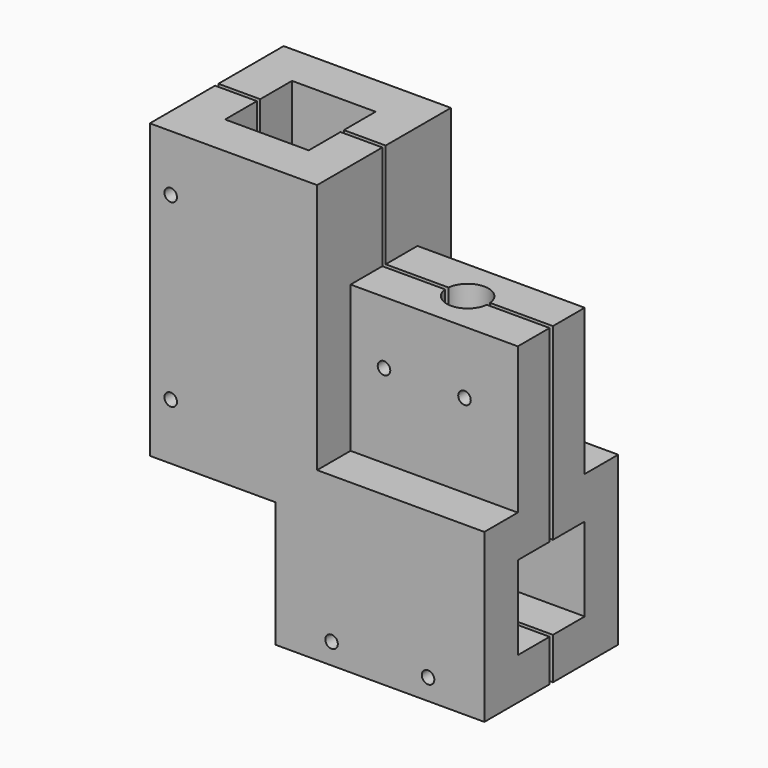
from build123d import *

# Parameters (mm, degrees)
F1_DEPTH        = 20
F2_W            = 50
F2_H            = 10
F3_DEPTH        = 10
F4_W            = 50
F4_H            = 10
F5_DEPTH        = 10
F6_W            = 50
F6_H            = 10
F7_DEPTH        = 30
F8_W            = 10
F8_H            = 10
F9_DEPTH        = 60
F10_W           = 10
F10_H           = 70
F11_DEPTH       = 30
F12_R           = 5
F13_DEPTH       = 15
F16_DEPTH       = 70
F17_T1_DEPTH    = 17.2150489639
F17_S1_T1_DEPTH = 10.5
F18_W           = 10
F18_H           = 70
F18_W_2         = 50
F18_H_2         = 10
F20_DEPTH       = 9.5
F19_W           = 10
F19_H           = 70
F19_W_2         = 50
F19_H_2         = 10
F21_DEPTH       = 9.5
F22_R           = 1.5
F23_DEPTH       = 20
F24_R           = 1.5
F25_DEPTH       = 20
F26_DEPTH       = 3
F28_R           = 1.5
F29_DEPTH       = 10
F27_R           = 1.5
F30_DEPTH       = 10
F31_DEPTH       = 3


# Not quite as in the source:
# - a fillet or chamfer that OpenCascade refuses, or shapes differently, is made with other operations: its cross-section is extruded or revolved along the edge and cut away or added


with BuildPart() as f1:
    # F0 (on Front) → F1 (new body)
    with BuildSketch(Plane.XZ):
        Polygon((-40, 89.1929870069), (-50, 89.1929870069), (-50, 19.1929870069), (0, 19.1929870069), (0, 64.1929870069), (-40, 64.1929870069), align=None)
    extrude(amount=F1_DEPTH)

    # F2 (on face) → F3 (join)
    with BuildSketch(Plane.XZ.offset(20)):
        with Locations((-25, 24.1929870069)):
            Rectangle(F2_W, F2_H)
    extrude(amount=F3_DEPTH)

    # F4 (on face) → F5 (join)
    with BuildSketch(Plane(origin=(0, 0, 0), x_dir=(-1, 0, 0), z_dir=(0, 1, 0))):
        with Locations((25, 24.1929870069)):
            Rectangle(F4_W, F4_H)
    extrude(amount=F5_DEPTH)

    # F6 (on face) → F7 (join)
    with BuildSketch(Plane(origin=(0, 0, 19.1929870069), x_dir=(1, 0, 0), z_dir=(0, 0, -1))):
        with Locations((-25, 25)):
            Rectangle(F6_W, F6_H)
        with Locations((-25, -5)):
            Rectangle(F6_W, F6_H)
    extrude(amount=F7_DEPTH)

    # F8 (on face) → F9 (join)
    with BuildSketch(Plane.XY.offset(29.1929870069)):
        with Locations((-45, 5)):
            Rectangle(F8_W, F8_H)
        with Locations((-45, -25)):
            Rectangle(F8_W, F8_H)
    extrude(amount=F9_DEPTH)

    # F10 (on face) → F11 (join)
    with BuildSketch(Plane(origin=(-50, 0, 0), x_dir=(0, -1, 0), z_dir=(-1, 0, 0))):
        with Locations((25, 54.1929870069)):
            Rectangle(F10_W, F10_H)
        with Locations((-5, 54.1929870069)):
            Rectangle(F10_W, F10_H)
    extrude(amount=F11_DEPTH)

    # F12 (on face) → F13 (cut)
    with BuildSketch(Plane.XY.offset(64.1929870069)):
        with Locations((-20, -10)):
            Circle(F12_R)
    extrude(amount=-F13_DEPTH, mode=Mode.SUBTRACT)

    # F15 (on face) + F14 (on face) → F16 (cut)
    with BuildSketch(Plane.XY.offset(64.1929870069)):
        with BuildLine():
            Line((0, -10.5), (0, -9.5))
            Line((0, -9.5), (-15.0250628145, -9.5))
            ThreePointArc((-15.0250628145, -9.5), (-15.0062696344, -9.7496861247), (-15, -10))
            ThreePointArc((-15, -10), (-15.0062696344, -10.2503138753), (-15.0250628145, -10.5))
            Line((-15.0250628145, -10.5), (0, -10.5))
        make_face()
        with BuildLine():
            Line((-15.0250628145, -9.5), (-24.9749371855, -9.5))
            ThreePointArc((-24.9749371855, -9.5), (-25, -10), (-24.9749371855, -10.5))
            Line((-24.9749371855, -10.5), (-15.0250628145, -10.5))
            ThreePointArc((-15.0250628145, -10.5), (-15.0062696344, -10.2503138753), (-15, -10))
            ThreePointArc((-15, -10), (-15.0062696344, -9.7496861247), (-15.0250628145, -9.5))
        make_face()
        with BuildLine():
            Line((-24.9749371855, -9.5), (-40, -9.5))
            Line((-40, -9.5), (-40, -10.5))
            Line((-40, -10.5), (-24.9749371855, -10.5))
            ThreePointArc((-24.9749371855, -10.5), (-25, -10), (-24.9749371855, -9.5))
        make_face()
    with BuildSketch(Plane.XY.offset(89.1929870069)):
        Polygon((-40, -10.5), (-40, -10), (-40, -9.5), (-50, -9.5), (-50, -10.5), align=None)
    extrude(amount=-F16_DEPTH, mode=Mode.SUBTRACT)

    # F17: chamfer of 3 on 1 edges, made by hand

    # F17_s2 → F17_t1 (cut)
    with BuildSketch(Plane.XZ.offset(2.7849510361)):
        Polygon((-47, 19.1929870069), (-50, 22.1929870069), (-50, 19.1929870069), align=None)
    extrude(amount=F17_T1_DEPTH, mode=Mode.SUBTRACT)

    # F17#s1: chamfer of 3 on 1 edges, made by hand

    # F17_s1_s2 → F17_s1_t1 (cut)
    with BuildSketch(Plane.XZ):
        Polygon((-50, 22.1929870069), (-47, 19.1929870069), (-50, 19.1929870069), align=None)
    extrude(amount=F17_S1_T1_DEPTH, mode=Mode.SUBTRACT)

    # F18 (on face) → F20 (join)
    with BuildSketch(Plane.XZ):
        with Locations((-75, 54.1929870069)):
            Rectangle(F18_W, F18_H)
        with Locations((-25, -5.8070129931)):
            Rectangle(F18_W_2, F18_H_2)
    extrude(amount=F20_DEPTH)

    # F19 (on face) → F21 (join)
    with BuildSketch(Plane(origin=(0, -20, 0), x_dir=(-1, 0, 0), z_dir=(0, 1, 0))):
        with Locations((75, 54.1929870069)):
            Rectangle(F19_W, F19_H)
        with Locations((25, -5.8070129931)):
            Rectangle(F19_W_2, F19_H_2)
    extrude(amount=F21_DEPTH)

    # F22 (on face) → F23 (cut)
    with BuildSketch(Plane.XZ.offset(30)):
        with Locations((-13.464, -5.8070129931)):
            Circle(F22_R)
        with Locations((-75, 75.7289870069)):
            Circle(F22_R)
        with Locations((-75, 32.6569870069)):
            Circle(F22_R)
        with Locations((-36.536, -5.8070129931)):
            Circle(F22_R)
    extrude(amount=-F23_DEPTH, mode=Mode.SUBTRACT)

    # F24 (on face) → F25 (cut)
    with BuildSketch(Plane(origin=(0, 10, 0), x_dir=(-1, 0, 0), z_dir=(0, 1, 0))):
        with Locations((13.4641016151, -5.8070129931)):
            Circle(F24_R)
        with Locations((36.5358983849, -5.8070129931)):
            Circle(F24_R)
        with Locations((75, 32.657088622)):
            Circle(F24_R)
        with Locations((75, 75.7288853918)):
            Circle(F24_R)
    extrude(amount=-F25_DEPTH, mode=Mode.SUBTRACT)

    # F24 (on face) → F26 (cut)
    with BuildSketch(Plane(origin=(0, 10, 0), x_dir=(-1, 0, 0), z_dir=(0, 1, 0))):
        Polygon((34.8038475773, -2.8070129931), (33.0717967697, -5.8070129931), (34.8038475773, -8.8070129931), (38.2679491924, -8.8070129931), (40, -5.8070129931), (38.2679491924, -2.8070129931), align=None)
        with Locations((36.5358983849, -5.8070129931)):
            Circle(F24_R, mode=Mode.SUBTRACT)
        Polygon((11.7320508076, -2.8070129931), (10, -5.8070129931), (11.7320508076, -8.8070129931), (15.1961524227, -8.8070129931), (16.9282032303, -5.8070129931), (15.1961524227, -2.8070129931), align=None)
        with Locations((13.4641016151, -5.8070129931)):
            Circle(F24_R, mode=Mode.SUBTRACT)
        Polygon((72, 30.9250378145), (75, 29.1929870069), (78, 30.9250378145), (78, 34.3891394296), (75, 36.1211902372), (72, 34.3891394296), align=None)
        with Locations((75, 32.657088622)):
            Circle(F24_R, mode=Mode.SUBTRACT)
        Polygon((72, 73.9968345842), (75, 72.2647837766), (78, 73.9968345842), (78, 77.4609361993), (75, 79.1929870069), (72, 77.4609361993), align=None)
        with Locations((75, 75.7288853918)):
            Circle(F24_R, mode=Mode.SUBTRACT)
    extrude(amount=-F26_DEPTH, mode=Mode.SUBTRACT)

    # F28 (on face) → F29 (cut)
    with BuildSketch(Plane(origin=(0, 0, 0), x_dir=(-1, 0, 0), z_dir=(0, 1, 0))):
        with Locations((32, 49.1929870069)):
            Circle(F28_R)
        with Locations((12.75, 49.1929870069)):
            Circle(F28_R)
    extrude(amount=-F29_DEPTH, mode=Mode.SUBTRACT)

    # F27 (on face) → F30 (cut)
    with BuildSketch(Plane.XZ.offset(20)):
        with Locations((-32, 49.1929870069)):
            Circle(F27_R)
        with Locations((-12.75, 49.1929870069)):
            Circle(F27_R)
    extrude(amount=-F30_DEPTH, mode=Mode.SUBTRACT)

    # F28 (on face) → F31 (cut)
    with BuildSketch(Plane(origin=(0, 0, 0), x_dir=(-1, 0, 0), z_dir=(0, 1, 0))):
        Polygon((30.2679491924, 52.1929870069), (28.5358983849, 49.1929870069), (30.2679491924, 46.1929870069), (33.7320508076, 46.1929870069), (35.4641016151, 49.1929870069), (33.7320508076, 52.1929870069), align=None)
        with Locations((32, 49.1929870069)):
            Circle(F28_R, mode=Mode.SUBTRACT)
        Polygon((11.0179491924, 52.1929870069), (9.2858983849, 49.1929870069), (11.0179491924, 46.1929870069), (14.4820508076, 46.1929870069), (16.2141016151, 49.1929870069), (14.4820508076, 52.1929870069), align=None)
        with Locations((12.75, 49.1929870069)):
            Circle(F28_R, mode=Mode.SUBTRACT)
    extrude(amount=-F31_DEPTH, mode=Mode.SUBTRACT)


solid = f1.part
